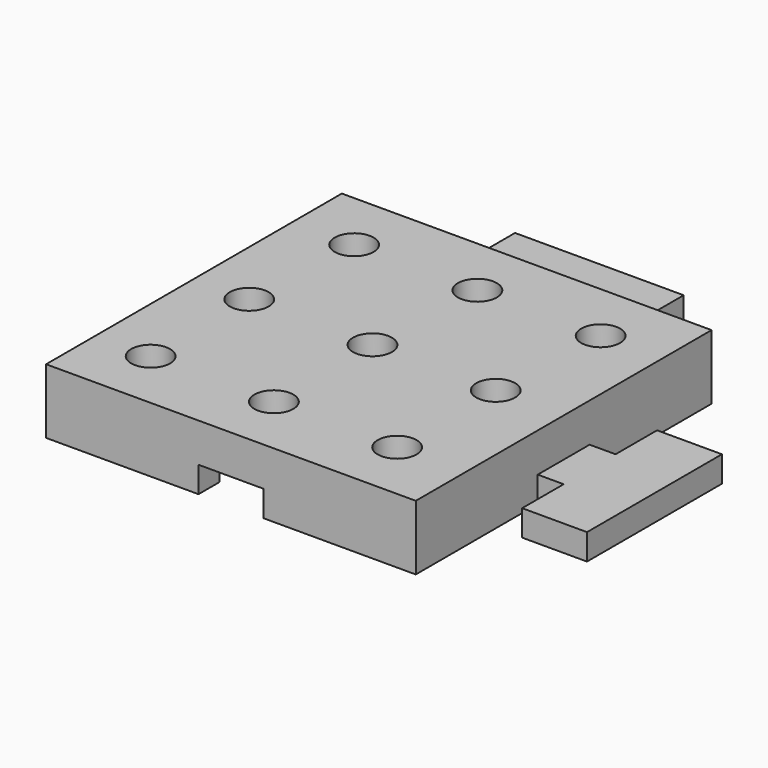
from build123d import *

# Parameters (mm, degrees)
F0_W     = 72.39
F0_H     = 72.39
F1_DEPTH = 12.7
F2_R     = 3.81
F3_DEPTH = 6.35
F5_DEPTH = 5.08
F7_DEPTH = 5.08
F8_W     = 4.1331201792
F8_H     = 7.04711047
F8_W_2   = 14.3668507226
F8_H_2   = 5.652282387
F9_DEPTH = 2.54


with BuildPart() as f1:
    # F0 (on Top) → F1 (new body)
    with BuildSketch(Plane.XY):
        with Locations((-36.195, -36.195)):
            Rectangle(F0_W, F0_H)
    extrude(amount=F1_DEPTH)

    # F2 (on face) → F3 (cut)
    with BuildSketch(Plane.XY.offset(12.7)):
        with Locations((-60.325, -12.065)):
            Circle(F2_R)
        with Locations((-61.5655786634, -36.195)):
            Circle(F2_R)
        with Locations((-61.5633073788, -60.325)):
            Circle(F2_R)
        with Locations((-36.195, -12.065)):
            Circle(F2_R)
        with Locations((-37.4355786634, -36.195)):
            Circle(F2_R)
        with Locations((-37.4333073788, -60.325)):
            Circle(F2_R)
        with Locations((-12.065, -12.065)):
            Circle(F2_R)
        with Locations((-13.3055786634, -36.195)):
            Circle(F2_R)
        with Locations((-13.3033073788, -60.325)):
            Circle(F2_R)
    extrude(amount=-F3_DEPTH, mode=Mode.SUBTRACT)

    # F4 (on face) → F5 (join)
    with BuildSketch(Plane(origin=(0, 0, 0), x_dir=(1, 0, 0), z_dir=(0, 0, -1))):
        Polygon((5.08, 42.545), (0, 42.545), (0, 29.845), (5.08, 29.845), (5.08, 19.685), (17.78, 19.685), (17.78, 52.705), (5.08, 52.705), align=None)
        Polygon((-29.845, -5.08), (-29.845, 0), (-42.545, 0), (-42.545, -5.08), (-52.705, -5.08), (-52.705, -17.78), (-19.685, -17.78), (-19.685, -5.08), align=None)
    extrude(amount=-F5_DEPTH)

    # F6 (on face) → F7 (cut)
    with BuildSketch(Plane(origin=(0, 0, 0), x_dir=(1, 0, 0), z_dir=(0, 0, -1))):
        Polygon((-44.1891504281, -29.484081471), (-56.8891504281, -29.484081471), (-56.8891504281, -42.184081471), (-44.1891504281, -42.184081471), (-44.1891504281, -54.884081471), (-31.4891504281, -54.884081471), (-31.4891504281, -17.78), (-44.1891504281, -17.78), align=None)
        Polygon((-72.39, 42.545), (-72.39, 29.845), (-67.31, 29.845), (-67.31, 19.685), (-54.61, 19.685), (-54.61, 52.705), (-67.31, 52.705), (-67.31, 42.545), align=None)
        Polygon((-29.845, 72.39), (-42.545, 72.39), (-42.545, 67.31), (-52.705, 67.31), (-52.705, 54.61), (-19.685, 54.61), (-19.685, 67.31), (-29.845, 67.31), align=None)
    extrude(amount=-F7_DEPTH, mode=Mode.SUBTRACT)

    # F8 (on face) → F9 (join)
    with BuildSketch(Plane(origin=(0, 0, 0), x_dir=(1, 0, 0), z_dir=(0, 0, -1))):
        with Locations((-36.4783331752, -0.2260982292)):
            Rectangle(F8_W, F8_H)
        with Locations((-3.0054978561, 35.1009014994)):
            Rectangle(F8_W_2, F8_H_2)
    extrude(amount=-F9_DEPTH)


solid = f1.part
